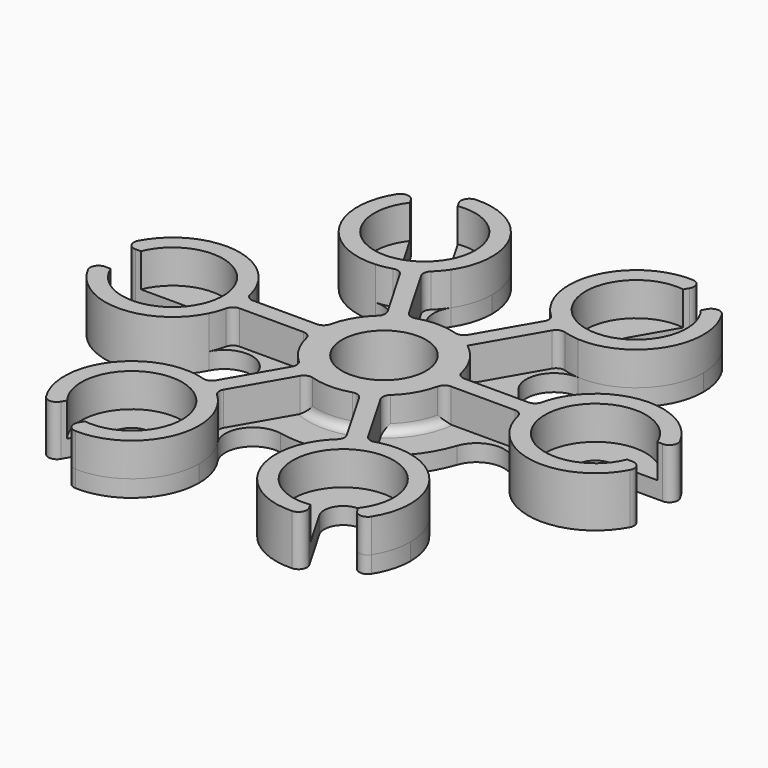
from build123d import *

# Parameters (mm, degrees)
F0_R     = 5
F1_DEPTH = 2
F2_R     = 5
F3_DEPTH = 4
F4_R     = 1


# Not quite as in the source:
# - a feature names something its author has since deleted; it is built from what else it names


with BuildPart() as f1:
    # F0 (on Top) → F1 (new body)
    with BuildSketch(Plane.XY):
        with BuildLine():
            Line((25.1463050069, 2.25), (32.8233812733, 2.25))
            ThreePointArc((32.8233812733, 2.25), (25.8365128088, 7.9701702109), (17.9703122908, 3.5362591166))
            ThreePointArc((17.9703122908, 3.5362591166), (17.1463050069, 0), (17.9703122908, -3.5362591166))
            ThreePointArc((17.9703122908, -3.5362591166), (25.8365128088, -7.9701702109), (32.8233812733, -2.25))
            Line((32.8233812733, -2.25), (25.1463050069, -2.25))
            ThreePointArc((25.1463050069, -2.25), (22.8963050069, 0), (25.1463050069, 2.25))
        make_face()
        with BuildLine():
            ThreePointArc((17.9703122908, -3.5362591166), (17.1463050069, 0), (17.9703122908, 3.5362591166))
            ThreePointArc((17.9703122908, 3.5362591166), (14.7748130521, 1.6962773546), (11.8585412256, 3.9528470752))
            ThreePointArc((11.8585412256, 3.9528470752), (12.3385932205, 2.0022780376), (12.5, 0))
            ThreePointArc((12.5, 0), (12.3385932205, -2.0022780376), (11.8585412256, -3.9528470752))
            ThreePointArc((11.8585412256, -3.9528470752), (14.7748130521, -1.6962773546), (17.9703122908, -3.5362591166))
        make_face()
        with BuildLine():
            ThreePointArc((12.5, 0), (12.3385932205, 2.0022780376), (11.8585412256, 3.9528470752))
            ThreePointArc((11.8585412256, 3.9528470752), (10.8253175473, 6.25), (9.3525365972, 8.2933744156))
            ThreePointArc((9.3525365972, 8.2933744156), (6.25, 10.8253175473), (2.5060046284, 12.2462214908))
            ThreePointArc((2.5060046284, 12.2462214908), (0, 12.5), (-2.5060046284, 12.2462214908))
            ThreePointArc((-2.5060046284, 12.2462214908), (-6.25, 10.8253175473), (-9.3525365972, 8.2933744156))
            ThreePointArc((-9.3525365972, 8.2933744156), (-10.8253175473, 6.25), (-11.8585412256, 3.9528470752))
            ThreePointArc((-11.8585412256, 3.9528470752), (-12.5, 0), (-11.8585412256, -3.9528470752))
            ThreePointArc((-11.8585412256, -3.9528470752), (-10.8253175473, -6.25), (-9.3525365972, -8.2933744156))
            ThreePointArc((-9.3525365972, -8.2933744156), (-6.25, -10.8253175473), (-2.5060046284, -12.2462214908))
            ThreePointArc((-2.5060046284, -12.2462214908), (0, -12.5), (2.5060046284, -12.2462214908))
            ThreePointArc((2.5060046284, -12.2462214908), (6.25, -10.8253175473), (9.3525365972, -8.2933744156))
            ThreePointArc((9.3525365972, -8.2933744156), (10.8253175473, -6.25), (11.8585412256, -3.9528470752))
            ThreePointArc((11.8585412256, -3.9528470752), (12.3385932205, -2.0022780376), (12.5, 0))
        make_face()
        Circle(F0_R, mode=Mode.SUBTRACT)
        with BuildLine():
            ThreePointArc((2.5060046284, 12.2462214908), (6.25, 10.8253175473), (9.3525365972, 8.2933744156))
            ThreePointArc((9.3525365972, 8.2933744156), (8.856425807, 11.9472247619), (12.0476463747, 13.7946173995))
            ThreePointArc((12.0476463747, 13.7946173995), (8.5731525034, 14.849135717), (5.9226659161, 17.3308765161))
            ThreePointArc((5.9226659161, 17.3308765161), (5.918387245, 13.6435021166), (2.5060046284, 12.2462214908))
        make_face()
        with BuildLine():
            ThreePointArc((-9.3525365972, 8.2933744156), (-6.25, 10.8253175473), (-2.5060046284, 12.2462214908))
            ThreePointArc((-2.5060046284, 12.2462214908), (-5.918387245, 13.6435021166), (-5.9226659161, 17.3308765161))
            ThreePointArc((-5.9226659161, 17.3308765161), (-8.5731525034, 14.849135717), (-12.0476463747, 13.7946173995))
            ThreePointArc((-12.0476463747, 13.7946173995), (-8.856425807, 11.9472247619), (-9.3525365972, 8.2933744156))
        make_face()
        with BuildLine():
            ThreePointArc((-11.8585412256, -3.9528470752), (-12.5, 0), (-11.8585412256, 3.9528470752))
            ThreePointArc((-11.8585412256, 3.9528470752), (-14.7748130521, 1.6962773546), (-17.9703122908, 3.5362591166))
            ThreePointArc((-17.9703122908, 3.5362591166), (-17.3550297028, 1.8154969391), (-17.1463050069, 0))
            ThreePointArc((-17.1463050069, 0), (-17.3550297028, -1.8154969391), (-17.9703122908, -3.5362591166))
            ThreePointArc((-17.9703122908, -3.5362591166), (-14.7748130521, -1.6962773546), (-11.8585412256, -3.9528470752))
        make_face()
        with BuildLine():
            ThreePointArc((-5.9226659161, -17.3308765161), (-5.918387245, -13.6435021166), (-2.5060046284, -12.2462214908))
            ThreePointArc((-2.5060046284, -12.2462214908), (-6.25, -10.8253175473), (-9.3525365972, -8.2933744156))
            ThreePointArc((-9.3525365972, -8.2933744156), (-8.856425807, -11.9472247619), (-12.0476463747, -13.7946173995))
            ThreePointArc((-12.0476463747, -13.7946173995), (-8.5731525034, -14.849135717), (-5.9226659161, -17.3308765161))
        make_face()
        with BuildLine():
            ThreePointArc((12.0476463747, -13.7946173995), (8.856425807, -11.9472247619), (9.3525365972, -8.2933744156))
            ThreePointArc((9.3525365972, -8.2933744156), (6.25, -10.8253175473), (2.5060046284, -12.2462214908))
            ThreePointArc((2.5060046284, -12.2462214908), (5.918387245, -13.6435021166), (5.9226659161, -17.3308765161))
            ThreePointArc((5.9226659161, -17.3308765161), (8.5731525034, -14.849135717), (12.0476463747, -13.7946173995))
        make_face()
        with BuildLine():
            ThreePointArc((20.5731525034, -21.7773389473), (18.0410566252, -15.9376450756), (12.0476463747, -13.7946173995))
            ThreePointArc((12.0476463747, -13.7946173995), (8.5731525034, -14.849135717), (5.9226659161, -17.3308765161))
            ThreePointArc((5.9226659161, -17.3308765161), (6.0158865293, -26.3601615431), (14.4631334781, -29.5508820207))
            Line((14.4631334781, -29.5508820207), (10.6245953449, -22.9023389473))
            ThreePointArc((10.6245953449, -22.9023389473), (11.4481525034, -19.8287817887), (14.5217096619, -20.6523389473))
            Line((14.5217096619, -20.6523389473), (18.3602477951, -27.3008820207))
            ThreePointArc((18.3602477951, -27.3008820207), (19.9993481086, -24.7525059734), (20.5731525034, -21.7773389473))
        make_face()
        with BuildLine():
            ThreePointArc((-4.5731525034, -21.7773389473), (-4.9179616927, -19.453967765), (-5.9226659161, -17.3308765161))
            ThreePointArc((-5.9226659161, -17.3308765161), (-8.5731525034, -14.849135717), (-12.0476463747, -13.7946173995))
            ThreePointArc((-12.0476463747, -13.7946173995), (-19.8206262795, -18.3899913322), (-18.3602477951, -27.3008820207))
            Line((-18.3602477951, -27.3008820207), (-14.5217096619, -20.6523389473))
            ThreePointArc((-14.5217096619, -20.6523389473), (-11.990809652, -19.6040058381), (-10.3231525034, -21.7773389473))
            ThreePointArc((-10.3231525034, -21.7773389473), (-10.3998193943, -22.3596817987), (-10.6245953449, -22.9023389473))
            Line((-10.6245953449, -22.9023389473), (-14.4631334781, -29.5508820207))
            ThreePointArc((-14.4631334781, -29.5508820207), (-7.6294619689, -28.067006975), (-4.5731525034, -21.7773389473))
        make_face()
        with BuildLine():
            ThreePointArc((-17.1463050069, 0), (-17.3550297028, 1.8154969391), (-17.9703122908, 3.5362591166))
            ThreePointArc((-17.9703122908, 3.5362591166), (-25.8365128088, 7.9701702109), (-32.8233812733, 2.25))
            Line((-32.8233812733, 2.25), (-25.1463050069, 2.25))
            ThreePointArc((-25.1463050069, 2.25), (-23.5553147492, 1.5909902577), (-22.8963050069, 0))
            ThreePointArc((-22.8963050069, 0), (-23.5553147492, -1.5909902577), (-25.1463050069, -2.25))
            Line((-25.1463050069, -2.25), (-32.8233812733, -2.25))
            ThreePointArc((-32.8233812733, -2.25), (-25.8365128088, -7.9701702109), (-17.9703122908, -3.5362591166))
            ThreePointArc((-17.9703122908, -3.5362591166), (-17.3550297028, -1.8154969391), (-17.1463050069, 0))
        make_face()
        with BuildLine():
            ThreePointArc((-12.0476463747, 13.7946173995), (-8.5731525034, 14.849135717), (-5.9226659161, 17.3308765161))
            ThreePointArc((-5.9226659161, 17.3308765161), (-4.9179616927, 19.453967765), (-4.5731525034, 21.7773389473))
            ThreePointArc((-4.5731525034, 21.7773389473), (-7.6294619689, 28.067006975), (-14.4631334781, 29.5508820207))
            Line((-14.4631334781, 29.5508820207), (-10.6245953449, 22.9023389473))
            ThreePointArc((-10.6245953449, 22.9023389473), (-10.3998193943, 22.3596817987), (-10.3231525034, 21.7773389473))
            ThreePointArc((-10.3231525034, 21.7773389473), (-11.990809652, 19.6040058381), (-14.5217096619, 20.6523389473))
            Line((-14.5217096619, 20.6523389473), (-18.3602477951, 27.3008820207))
            ThreePointArc((-18.3602477951, 27.3008820207), (-19.8206262795, 18.3899913322), (-12.0476463747, 13.7946173995))
        make_face()
        with BuildLine():
            ThreePointArc((5.9226659161, 17.3308765161), (8.5731525034, 14.849135717), (12.0476463747, 13.7946173995))
            ThreePointArc((12.0476463747, 13.7946173995), (18.0410566252, 15.9376450756), (20.5731525034, 21.7773389473))
            ThreePointArc((20.5731525034, 21.7773389473), (19.9993481086, 24.7525059734), (18.3602477951, 27.3008820207))
            Line((18.3602477951, 27.3008820207), (14.5217096619, 20.6523389473))
            ThreePointArc((14.5217096619, 20.6523389473), (11.4481525034, 19.8287817887), (10.6245953449, 22.9023389473))
            Line((10.6245953449, 22.9023389473), (14.4631334781, 29.5508820207))
            ThreePointArc((14.4631334781, 29.5508820207), (6.0158865293, 26.3601615431), (5.9226659161, 17.3308765161))
        make_face()
    extrude(amount=F1_DEPTH)

    # F2 (on face) → F3 (join)
    with BuildSketch(Plane.XY.offset(2)):
        with BuildLine():
            Line((7.9372539332, -1), (17.2090510737, -1))
            ThreePointArc((17.2090510737, -1), (17.1463050069, 0), (17.2090510737, 1))
            Line((17.2090510737, 1), (7.9372539332, 1))
            ThreePointArc((7.9372539332, 1), (7.9842980739, 0.5009833003), (8, 0))
            ThreePointArc((8, 0), (7.9842980739, -0.5009833003), (7.9372539332, -1))
        make_face()
        with BuildLine():
            ThreePointArc((17.9703122908, -3.5362591166), (25.8365128088, -7.9701702109), (32.8233812733, -2.25))
            Line((32.8233812733, -2.25), (30.7084538722, -2.25))
            ThreePointArc((30.7084538722, -2.25), (19.1463050069, 0), (30.7084538722, 2.25))
            Line((30.7084538722, 2.25), (32.8233812733, 2.25))
            ThreePointArc((32.8233812733, 2.25), (25.8365128088, 7.9701702109), (17.9703122908, 3.5362591166))
            ThreePointArc((17.9703122908, 3.5362591166), (17.4840136625, 2.2998459412), (17.2090510737, 1))
            ThreePointArc((17.2090510737, 1), (17.1463050069, 0), (17.2090510737, -1))
            ThreePointArc((17.2090510737, -1), (17.4840136625, -2.2998459412), (17.9703122908, -3.5362591166))
        make_face()
        with BuildLine():
            ThreePointArc((4.8346523704, -6.3738635424), (6.9282032303, -4), (7.9372539332, -1))
            ThreePointArc((7.9372539332, -1), (7.9842980739, -0.5009833003), (8, 0))
            ThreePointArc((8, 0), (7.9842980739, 0.5009833003), (7.9372539332, 1))
            ThreePointArc((7.9372539332, 1), (6.9282032303, 4), (4.8346523704, 6.3738635424))
            ThreePointArc((4.8346523704, 6.3738635424), (4, 6.9282032303), (3.1026015628, 7.3738635424))
            ThreePointArc((3.1026015628, 7.3738635424), (0, 8), (-3.1026015628, 7.3738635424))
            ThreePointArc((-3.1026015628, 7.3738635424), (-4, 6.9282032303), (-4.8346523704, 6.3738635424))
            ThreePointArc((-4.8346523704, 6.3738635424), (-6.9282032303, 4), (-7.9372539332, 1))
            ThreePointArc((-7.9372539332, 1), (-8, 0), (-7.9372539332, -1))
            ThreePointArc((-7.9372539332, -1), (-6.9282032303, -4), (-4.8346523704, -6.3738635424))
            ThreePointArc((-4.8346523704, -6.3738635424), (-4, -6.9282032303), (-3.1026015628, -7.3738635424))
            ThreePointArc((-3.1026015628, -7.3738635424), (0, -8), (3.1026015628, -7.3738635424))
            ThreePointArc((3.1026015628, -7.3738635424), (4, -6.9282032303), (4.8346523704, -6.3738635424))
        make_face()
        Circle(F2_R, mode=Mode.SUBTRACT)
        with BuildLine():
            Line((9.4705509406, -14.4034754048), (4.8346523704, -6.3738635424))
            ThreePointArc((4.8346523704, -6.3738635424), (4, -6.9282032303), (3.1026015628, -7.3738635424))
            Line((3.1026015628, -7.3738635424), (7.7385001331, -15.4034754048))
            ThreePointArc((7.7385001331, -15.4034754048), (8.5731525034, -14.849135717), (9.4705509406, -14.4034754048))
        make_face()
        with BuildLine():
            ThreePointArc((18.3602477951, -27.3008820207), (19.8206262795, -18.3899913322), (12.0476463747, -13.7946173995))
            ThreePointArc((12.0476463747, -13.7946173995), (10.7337318411, -13.9916770212), (9.4705509406, -14.4034754048))
            ThreePointArc((9.4705509406, -14.4034754048), (8.5731525034, -14.849135717), (7.7385001331, -15.4034754048))
            ThreePointArc((7.7385001331, -15.4034754048), (6.7502818213, -16.2915229624), (5.9226659161, -17.3308765161))
            ThreePointArc((5.9226659161, -17.3308765161), (6.0158865293, -26.3601615431), (14.4631334781, -29.5508820207))
            Line((14.4631334781, -29.5508820207), (13.4056697776, -27.7193011643))
            ThreePointArc((13.4056697776, -27.7193011643), (9.5731525034, -16.5811865246), (17.3027840946, -25.4693011643))
            Line((17.3027840946, -25.4693011643), (18.3602477951, -27.3008820207))
        make_face()
        with BuildLine():
            ThreePointArc((-5.9226659161, -17.3308765161), (-6.7502818213, -16.2915229624), (-7.7385001331, -15.4034754048))
            ThreePointArc((-7.7385001331, -15.4034754048), (-8.5731525034, -14.849135717), (-9.4705509406, -14.4034754048))
            ThreePointArc((-9.4705509406, -14.4034754048), (-10.7337318411, -13.9916770212), (-12.0476463747, -13.7946173995))
            ThreePointArc((-12.0476463747, -13.7946173995), (-19.8206262795, -18.3899913322), (-18.3602477951, -27.3008820207))
            Line((-18.3602477951, -27.3008820207), (-17.3027840946, -25.4693011643))
            ThreePointArc((-17.3027840946, -25.4693011643), (-9.5731525034, -16.5811865246), (-13.4056697776, -27.7193011643))
            Line((-13.4056697776, -27.7193011643), (-14.4631334781, -29.5508820207))
            ThreePointArc((-14.4631334781, -29.5508820207), (-6.0158865293, -26.3601615431), (-5.9226659161, -17.3308765161))
        make_face()
        with BuildLine():
            Line((-7.7385001331, -15.4034754048), (-3.1026015628, -7.3738635424))
            ThreePointArc((-3.1026015628, -7.3738635424), (-4, -6.9282032303), (-4.8346523704, -6.3738635424))
            Line((-4.8346523704, -6.3738635424), (-9.4705509406, -14.4034754048))
            ThreePointArc((-9.4705509406, -14.4034754048), (-8.5731525034, -14.849135717), (-7.7385001331, -15.4034754048))
        make_face()
        with BuildLine():
            Line((-17.2090510737, -1), (-7.9372539332, -1))
            ThreePointArc((-7.9372539332, -1), (-8, 0), (-7.9372539332, 1))
            Line((-7.9372539332, 1), (-17.2090510737, 1))
            ThreePointArc((-17.2090510737, 1), (-17.1463050069, 0), (-17.2090510737, -1))
        make_face()
        with BuildLine():
            ThreePointArc((-17.9703122908, -3.5362591166), (-17.4840136625, -2.2998459412), (-17.2090510737, -1))
            ThreePointArc((-17.2090510737, -1), (-17.1463050069, 0), (-17.2090510737, 1))
            ThreePointArc((-17.2090510737, 1), (-17.4840136625, 2.2998459412), (-17.9703122908, 3.5362591166))
            ThreePointArc((-17.9703122908, 3.5362591166), (-25.8365128088, 7.9701702109), (-32.8233812733, 2.25))
            Line((-32.8233812733, 2.25), (-30.7084538722, 2.25))
            ThreePointArc((-30.7084538722, 2.25), (-19.1463050069, 0), (-30.7084538722, -2.25))
            Line((-30.7084538722, -2.25), (-32.8233812733, -2.25))
            ThreePointArc((-32.8233812733, -2.25), (-25.8365128088, -7.9701702109), (-17.9703122908, -3.5362591166))
        make_face()
        with BuildLine():
            ThreePointArc((-9.4705509406, 14.4034754048), (-8.5731525034, 14.849135717), (-7.7385001331, 15.4034754048))
            ThreePointArc((-7.7385001331, 15.4034754048), (-6.7502818213, 16.2915229624), (-5.9226659161, 17.3308765161))
            ThreePointArc((-5.9226659161, 17.3308765161), (-6.0158865293, 26.3601615431), (-14.4631334781, 29.5508820207))
            Line((-14.4631334781, 29.5508820207), (-13.4056697776, 27.7193011643))
            ThreePointArc((-13.4056697776, 27.7193011643), (-9.5731525034, 16.5811865246), (-17.3027840946, 25.4693011643))
            Line((-17.3027840946, 25.4693011643), (-18.3602477951, 27.3008820207))
            ThreePointArc((-18.3602477951, 27.3008820207), (-19.8206262795, 18.3899913322), (-12.0476463747, 13.7946173995))
            ThreePointArc((-12.0476463747, 13.7946173995), (-10.7337318411, 13.9916770212), (-9.4705509406, 14.4034754048))
        make_face()
        with BuildLine():
            ThreePointArc((-4.8346523704, 6.3738635424), (-4, 6.9282032303), (-3.1026015628, 7.3738635424))
            Line((-3.1026015628, 7.3738635424), (-7.7385001331, 15.4034754048))
            ThreePointArc((-7.7385001331, 15.4034754048), (-8.5731525034, 14.849135717), (-9.4705509406, 14.4034754048))
            Line((-9.4705509406, 14.4034754048), (-4.8346523704, 6.3738635424))
        make_face()
        with BuildLine():
            ThreePointArc((3.1026015628, 7.3738635424), (4, 6.9282032303), (4.8346523704, 6.3738635424))
            Line((4.8346523704, 6.3738635424), (9.4705509406, 14.4034754048))
            ThreePointArc((9.4705509406, 14.4034754048), (8.5731525034, 14.849135717), (7.7385001331, 15.4034754048))
            Line((7.7385001331, 15.4034754048), (3.1026015628, 7.3738635424))
        make_face()
        with BuildLine():
            ThreePointArc((7.7385001331, 15.4034754048), (8.5731525034, 14.849135717), (9.4705509406, 14.4034754048))
            ThreePointArc((9.4705509406, 14.4034754048), (10.7337318411, 13.9916770212), (12.0476463747, 13.7946173995))
            ThreePointArc((12.0476463747, 13.7946173995), (19.8206262795, 18.3899913322), (18.3602477951, 27.3008820207))
            Line((18.3602477951, 27.3008820207), (17.3027840946, 25.4693011643))
            ThreePointArc((17.3027840946, 25.4693011643), (9.5731525034, 16.5811865246), (13.4056697776, 27.7193011643))
            Line((13.4056697776, 27.7193011643), (14.4631334781, 29.5508820207))
            ThreePointArc((14.4631334781, 29.5508820207), (6.0158865293, 26.3601615431), (5.9226659161, 17.3308765161))
            ThreePointArc((5.9226659161, 17.3308765161), (6.7502818213, 16.2915229624), (7.7385001331, 15.4034754048))
        make_face()
    extrude(amount=F3_DEPTH)

    # F4
    f4_edges = [f1.edges().sort_by_distance(p)[0] for p in [
        (32.823381, 2.25, 3),
        (32.823381, -2.25, 3),
        (14.463133, 29.550882, 3),
        (-18.360248, 27.300882, 3),
        (18.360248, 27.300882, 3),
        (-14.463133, 29.550882, 3),
        (-32.823381, 2.25, 3),
        (-32.823381, -2.25, 3),
        (-18.360248, -27.300882, 3),
        (-14.463133, -29.550882, 3),
        (14.463133, -29.550882, 3),
        (18.360248, -27.300882, 3),
        (4.834652, -6.373864, 4),
        (-7.7385, -15.403475, 4),
        (-17.209051, -1, 4),
        (-7.937254, 1, 4),
        (3.102602, 7.373864, 4),
        (17.209051, 1, 4),
        (-9.470551, -14.403475, 4),
        (-17.209051, 1, 4),
        (-9.470551, 14.403475, 4),
        (-7.7385, 15.403475, 4),
        (-3.102602, 7.373864, 4),
        (7.937254, 1, 4),
        (9.470551, -14.403475, 4),
        (17.209051, -1, 4),
        (7.7385, -15.403475, 4),
        (-4.834652, -6.373864, 4),
        (-3.102602, -7.373864, 4),
        (-4.834652, 6.373864, 4),
        (7.7385, 15.403475, 4),
        (9.470551, 14.403475, 4),
        (3.102602, -7.373864, 4),
        (7.937254, -1, 4),
        (-7.937254, -1, 4),
        (6.928203, 4, 2),
        (0, 8, 2),
        (-6.928203, 4, 2),
        (-6.928203, -4, 2),
        (0, -8, 2),
        (6.928203, -4, 2),
    ]]
    fillet(f4_edges, radius=F4_R)


solid = f1.part
